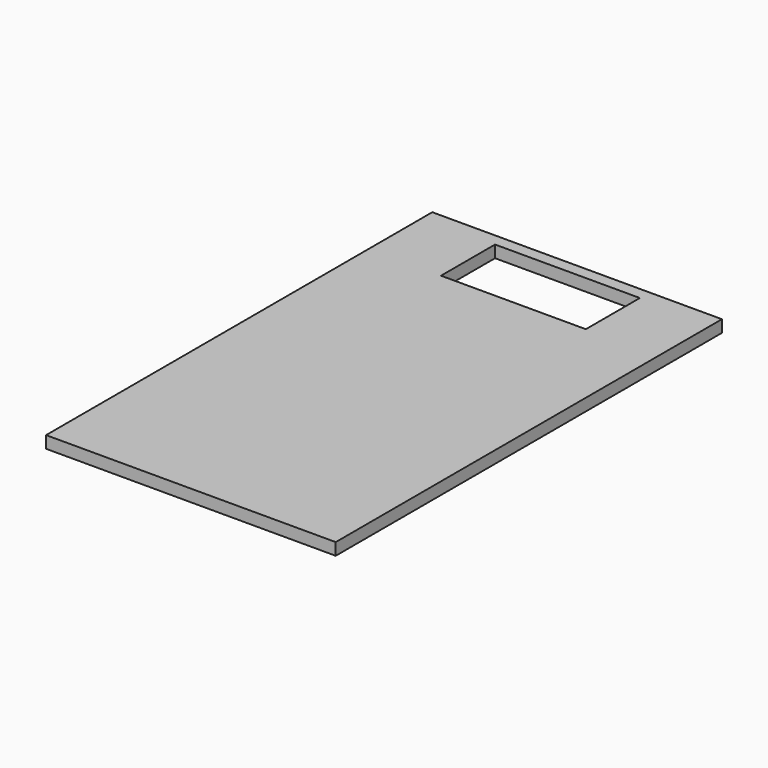
from build123d import *

# Parameters (mm, degrees)
F0_W     = 76.2
F0_H     = 127
F1_DEPTH = 3.175
F2_W     = 38.1
F2_H     = 17.7633663237
F3_DEPTH = 3.175


# Not quite as in the source:
# - a length typed as a fraction of an inch, garbled in the dataset ("3 / 203.2 mm" for 3/8 in), is restored


with BuildPart() as f1:
    # F0 (on Top) → F1 (new body)
    with BuildSketch(Plane.XY):
        with Locations((-7.4443402648, 10.8384059966)):
            Rectangle(F0_W, F0_H)
    extrude(amount=F1_DEPTH)

    # F2 (on face) → F3 (cut)
    with BuildSketch(Plane(origin=(0, 0, 0), x_dir=(1, 0, 0), z_dir=(0, 0, -1))):
        with Locations((-7.4443402648, -62.2817228347)):
            Rectangle(F2_W, F2_H)
    extrude(amount=-F3_DEPTH, mode=Mode.SUBTRACT)


solid = f1.part
